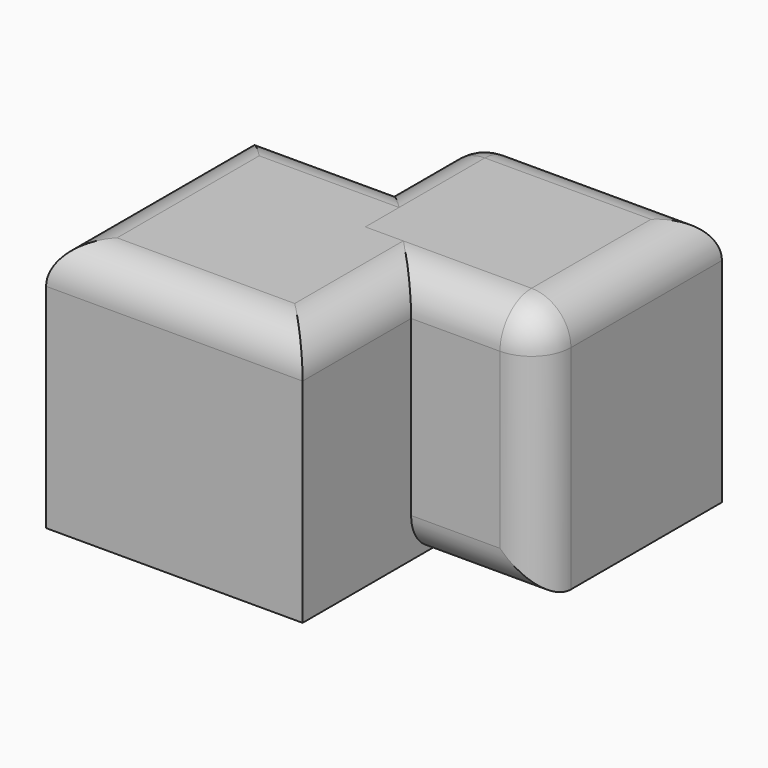
from build123d import *

# Parameters (mm, degrees)
F1_W        = 32.5374016538
F1_H        = 32.5373997912
F2_DEPTH    = 32
F0_W        = 31.0705509037
F0_H        = 28.9369504899
F3_R        = 5
F4_R        = 5
F5_T1_DEPTH = 48.9369504899
F5_T3_DEPTH = 39.5
F5_T5_DEPTH = 31.4369504899
F5_T8_ANGLE = 90
F6_R        = 5


# Not quite as in the source:
# - a fillet or chamfer that OpenCascade refuses, or shapes differently, is made with other operations: its cross-section is extruded or revolved along the edge and cut away or added


with BuildPart() as f2:
    # F1 (on Top) → F2 (new body)
    with BuildSketch(Plane.XY):
        with Locations((-1.4668493532, -0.933450181)):
            Rectangle(F1_W, F1_H)
    extrude(amount=F2_DEPTH)

    # F6
    f6_edges = [f2.edges().sort_by_distance(p)[0] for p in [
        (-1.466849, -17.20215, 32),
        (-17.73555, -0.93345, 32),
        (-1.466849, 15.33525, 32),
        (14.801851, -0.93345, 32),
    ]]
    fillet(f6_edges, radius=F6_R)


with BuildPart() as f2b:
    # F0 (on Top) → F2, piece 2 (new body)
    with BuildSketch(Plane.XY):
        with Locations((15.5352754518, 14.4684752449)):
            Rectangle(F0_W, F0_H)
    extrude(amount=F2_DEPTH)

    # F3
    f3_edges = [f2b.edges().sort_by_distance(p)[0] for p in [
        (15.535275, 28.93695, 32),
        (31.070551, 14.468475, 32),
    ]]
    fillet(f3_edges, radius=F3_R)

    # F4
    f4_edges = [f2b.edges().sort_by_distance(p)[0] for p in [
        (31.070551, 0, 13.5),
        (29.606085, 0, 30.535534),
        (15.535275, 0, 0),
        (13.035275, 0, 32),
        (0, 0, 16),
    ]]
    fillet(f4_edges, radius=F4_R)

    # F5: fillet of radius 5 on 5 edges, made by hand

    # F5_s2 → F5_t1 (cut)
    with BuildSketch(Plane.XZ.offset(-41.4369504899)):
        with BuildLine():
            ThreePointArc((0, 5), (1.4644660941, 1.4644660941), (5, 0))
            Line((5, 0), (0, 0))
            Line((0, 0), (0, 5))
        make_face()
    extrude(amount=F5_T1_DEPTH, mode=Mode.SUBTRACT)

    # F5_s4 → F5_t3 (cut)
    with BuildSketch(Plane.XY.offset(-12.5)):
        with BuildLine():
            ThreePointArc((0, 23.9369504899), (1.4644660941, 27.4724843958), (5, 28.9369504899))
            Line((5, 28.9369504899), (0, 28.9369504899))
            Line((0, 28.9369504899), (0, 23.9369504899))
        make_face()
    extrude(amount=F5_T3_DEPTH, mode=Mode.SUBTRACT)

    # F5_s6 → F5_t5 (cut)
    with BuildSketch(Plane.XZ.offset(-23.9369504899)):
        with BuildLine():
            ThreePointArc((0, 27), (1.4644660941, 30.5355339059), (5, 32))
            Line((5, 32), (0, 32))
            Line((0, 32), (0, 27))
        make_face()
    extrude(amount=F5_T5_DEPTH, mode=Mode.SUBTRACT)

    # F5_s7 → F5_t8 (revolve, cut)
    with BuildSketch(Plane.XY.offset(27)):
        with BuildLine():
            ThreePointArc((0, 23.9369504899), (1.4644660941, 27.4724843958), (5, 28.9369504899))
            Line((5, 28.9369504899), (0, 28.9369504899))
            Line((0, 28.9369504899), (0, 23.9369504899))
        make_face()
    revolve(axis=Axis((0, 23.9369504899, 27), (1, 0, 0)), revolution_arc=F5_T8_ANGLE, mode=Mode.SUBTRACT)


solid = Compound([f2.part, f2b.part])
